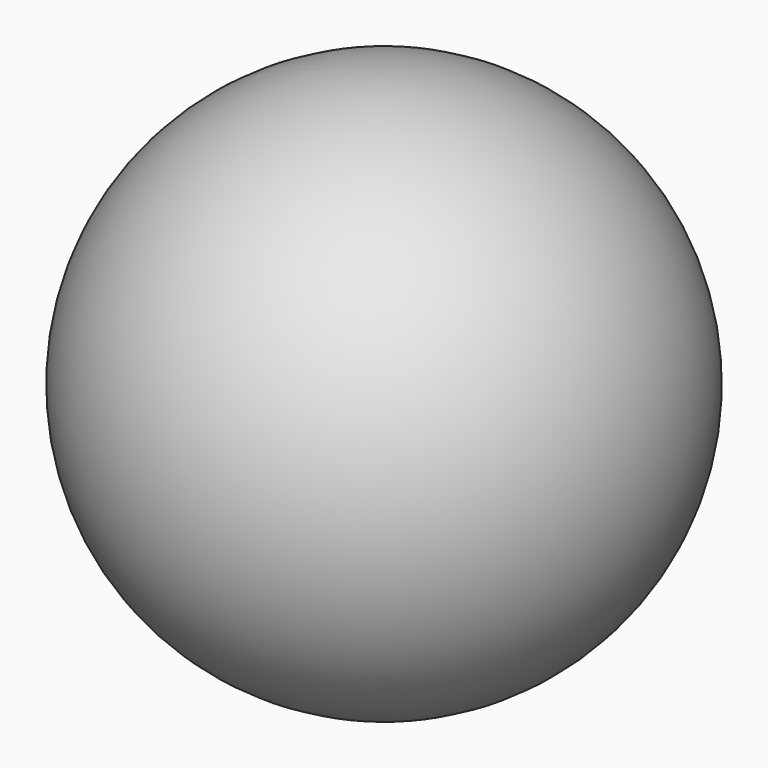
from build123d import *


with BuildPart() as f1:
    # F0 (on Front) → F1 (revolve)
    with BuildSketch(Plane.XZ):
        with BuildLine():
            Line((0, 0), (0, 6.35586852))
            ThreePointArc((0, 6.35586852), (-6.35586852, 0), (0, -6.35586852))
            Line((0, -6.35586852), (0, 0))
        make_face()
    revolve(axis=Axis((0, 0, 0), (0, 0, -1)))


solid = f1.part
